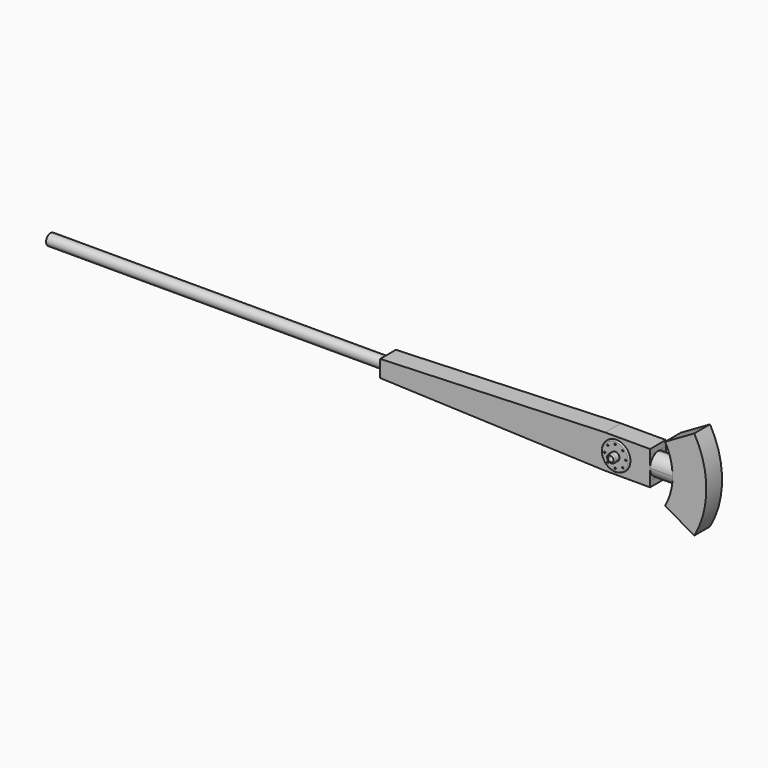
from build123d import *

# Parameters (mm, degrees)
F1_R          = 12.7
F2_DEPTH      = 88.9
F4_DEPTH      = 152.4
F5_R          = 25.4
F5_R_2        = 23.8125
F6_DEPTH      = 1524
F7_R          = 63.5
F7_R_2        = 3.175
F7_R_3        = 12.7
F8_DEPTH      = 6.35
F9_R          = 19.05
F9_R_2        = 12.7
F10_DEPTH     = 25.4
F11_R         = 5.08
F12_R         = 63.5
F12_R_2       = 3.175
F12_R_3       = 12.7
F13_DEPTH     = 6.35
F14_R         = 19.05
F14_R_2       = 12.7
F15_DEPTH     = 25.4
F16_R         = 5.08
F17_T4_DEPTH  = 222.8331578668
F17_S5_R      = 254
F17_T6_DEPTH  = 119
F17_T10_DEPTH = 222.8331578668
F17_S11_R     = 254
F17_T12_DEPTH = 119
F17_T16_DEPTH = 222.8331578668
F17_S17_R     = 254
F17_T18_DEPTH = 119
F17_T22_DEPTH = 222.8331578668
F17_S23_R     = 254
F17_T24_DEPTH = 119


# Not quite as in the source:
# - a fillet or chamfer that OpenCascade refuses, or shapes differently, is made with other operations: its cross-section is extruded or revolved along the edge and cut away or added


with BuildPart() as f2:
    # F1 (on Front) → F2 (new body)
    with BuildSketch(Plane.XZ):
        with BuildLine():
            Line((0, 76.2), (0, -76.2))
            Line((0, -76.2), (1219.2, -76.2))
            Line((1219.2, -76.2), (1219.2, -50.8))
            Line((1219.2, -50.8), (1315.6681578668, -50.8))
            ThreePointArc((1315.6681578668, -50.8), (1304.2953066, -90.0665273172), (1286.7704525612, -127))
            Line((1286.7704525612, -127), (1418.752724098, -203.2))
            ThreePointArc((1418.752724098, -203.2), (1473.2, 0), (1418.752724098, 203.2))
            Line((1418.752724098, 203.2), (1286.7704525612, 127))
            ThreePointArc((1286.7704525612, 127), (1304.2953066, 90.0665273172), (1315.6681578668, 50.8))
            Line((1315.6681578668, 50.8), (1219.2, 50.8))
            Line((1219.2, 50.8), (1219.2, 76.2))
            Line((1219.2, 76.2), (0, 76.2))
        make_face()
        with Locations((1066.8, 0)):
            Circle(F1_R, mode=Mode.SUBTRACT)
    extrude(amount=F2_DEPTH)

    # F3 (on face) → F4 (cut)
    with BuildSketch(Plane.XZ.offset(88.9)):
        Polygon((1016, 76.2), (0, 76.2), (0, 38.1), align=None)
        Polygon((0, -38.1), (0, -76.2), (1016, -76.2), align=None)
    extrude(amount=-F4_DEPTH, mode=Mode.SUBTRACT)

    # F5 (on face) → F6 (join)
    with BuildSketch(Plane(origin=(0, 0, 0), x_dir=(0, -1, 0), z_dir=(-1, 0, 0))):
        with Locations((44.45, 0)):
            Circle(F5_R)
        with Locations((44.45, 0)):
            Circle(F5_R_2, mode=Mode.SUBTRACT)
    extrude(amount=F6_DEPTH)

    # F7 (on face) → F8 (join)
    with BuildSketch(Plane.XZ.offset(88.9)):
        with Locations((1066.8, 0)):
            Circle(F7_R)
        with Locations((1033.124039546, -33.675960454)):
            Circle(F7_R_2, mode=Mode.SUBTRACT)
        with Locations((1066.8, -47.625)):
            Circle(F7_R_2, mode=Mode.SUBTRACT)
        with Locations((1100.475960454, -33.675960454)):
            Circle(F7_R_2, mode=Mode.SUBTRACT)
        with Locations((1019.175, 0)):
            Circle(F7_R_2, mode=Mode.SUBTRACT)
        with Locations((1033.124039546, 33.675960454)):
            Circle(F7_R_2, mode=Mode.SUBTRACT)
        with Locations((1066.8, 0)):
            Circle(F7_R_3, mode=Mode.SUBTRACT)
        with Locations((1114.425, 0)):
            Circle(F7_R_2, mode=Mode.SUBTRACT)
        with Locations((1066.8, 47.625)):
            Circle(F7_R_2, mode=Mode.SUBTRACT)
        with Locations((1100.475960454, 33.675960454)):
            Circle(F7_R_2, mode=Mode.SUBTRACT)
    extrude(amount=F8_DEPTH)

    # F9 (on face) → F10 (join)
    with BuildSketch(Plane.XZ.offset(95.25)):
        with Locations((1066.8, 0)):
            Circle(F9_R)
        with Locations((1066.8, 0)):
            Circle(F9_R_2, mode=Mode.SUBTRACT)
    extrude(amount=F10_DEPTH)

    # F11
    f11_edges = [f2.edges().sort_by_distance(p)[0] for p in [
        (1047.75, -120.65, 0),
        (1003.3, -95.25, 0),
    ]]
    fillet(f11_edges, radius=F11_R)

    # F12 (on face) → F13 (join)
    with BuildSketch(Plane(origin=(0, 0, 0), x_dir=(-1, 0, 0), z_dir=(0, 1, 0))):
        with Locations((-1066.8, 0)):
            Circle(F12_R)
        with Locations((-1100.475960454, -33.675960454)):
            Circle(F12_R_2, mode=Mode.SUBTRACT)
        with Locations((-1066.8, -47.625)):
            Circle(F12_R_2, mode=Mode.SUBTRACT)
        with Locations((-1033.124039546, -33.675960454)):
            Circle(F12_R_2, mode=Mode.SUBTRACT)
        with Locations((-1114.425, 0)):
            Circle(F12_R_2, mode=Mode.SUBTRACT)
        with Locations((-1100.475960454, 33.675960454)):
            Circle(F12_R_2, mode=Mode.SUBTRACT)
        with Locations((-1066.8, 0)):
            Circle(F12_R_3, mode=Mode.SUBTRACT)
        with Locations((-1019.175, 0)):
            Circle(F12_R_2, mode=Mode.SUBTRACT)
        with Locations((-1066.8, 47.625)):
            Circle(F12_R_2, mode=Mode.SUBTRACT)
        with Locations((-1033.124039546, 33.675960454)):
            Circle(F12_R_2, mode=Mode.SUBTRACT)
    extrude(amount=F13_DEPTH)

    # F14 (on face) → F15 (join)
    with BuildSketch(Plane(origin=(0, 6.35, 0), x_dir=(-1, 0, 0), z_dir=(0, 1, 0))):
        with Locations((-1066.8, 0)):
            Circle(F14_R)
        with Locations((-1066.8, 0)):
            Circle(F14_R_2, mode=Mode.SUBTRACT)
    extrude(amount=F15_DEPTH)

    # F16
    f16_edges = [f2.edges().sort_by_distance(p)[0] for p in [
        (1130.3, 6.35, 0),
        (1085.85, 31.75, 0),
    ]]
    fillet(f16_edges, radius=F16_R)

    # F17: fillet of radius 50.546 on 4 edges, made by hand


with BuildPart() as f17_tool2:
    # F17_s3 → F17_t4 (new body)
    with BuildSketch(Plane.YZ.offset(1442.0331578668)):
        with BuildLine():
            ThreePointArc((-38.354, 50.8), (-74.0954193619, 35.9954193619), (-88.9, 0.254))
            Line((-88.9, 0.254), (-88.9, 50.8))
            Line((-88.9, 50.8), (-38.354, 50.8))
        make_face()
    extrude(amount=-F17_T4_DEPTH)

    # F17_s5 → F17_t6 (intersect, symmetric)
    with BuildSketch(Plane.XZ.offset(63.6)):
        with Locations((1066.8, 0)):
            Circle(F17_S5_R)
    extrude(amount=F17_T6_DEPTH, both=True, mode=Mode.INTERSECT)


with BuildPart() as f2_1:
    add(f2.part)

    # F17_t1: cut F17_tool2
    add(f17_tool2.part, mode=Mode.SUBTRACT)


with BuildPart() as f17_tool8:
    # F17_s9 → F17_t10 (new body)
    with BuildSketch(Plane.YZ.offset(1219.2)):
        with BuildLine():
            ThreePointArc((-38.354, -50.8), (-74.0954193619, -35.9954193619), (-88.9, -0.254))
            Line((-88.9, -0.254), (-88.9, -50.8))
            Line((-88.9, -50.8), (-38.354, -50.8))
        make_face()
    extrude(amount=F17_T10_DEPTH)

    # F17_s11 → F17_t12 (intersect, symmetric)
    with BuildSketch(Plane.XZ.offset(63.6)):
        with Locations((1066.8, 0)):
            Circle(F17_S11_R)
    extrude(amount=F17_T12_DEPTH, both=True, mode=Mode.INTERSECT)


with BuildPart() as f2_2:
    add(f2_1.part)

    # F17_t7: cut F17_tool8
    add(f17_tool8.part, mode=Mode.SUBTRACT)


with BuildPart() as f17_tool14:
    # F17_s15 → F17_t16 (new body)
    with BuildSketch(Plane.YZ.offset(1219.2)):
        with BuildLine():
            ThreePointArc((0, -0.254), (-14.8045806381, -35.9954193619), (-50.546, -50.8))
            Line((-50.546, -50.8), (0, -50.8))
            Line((0, -50.8), (0, -0.254))
        make_face()
    extrude(amount=F17_T16_DEPTH)

    # F17_s17 → F17_t18 (intersect, symmetric)
    with BuildSketch(Plane.XZ.offset(25.3)):
        with Locations((1066.8, 0)):
            Circle(F17_S17_R)
    extrude(amount=F17_T18_DEPTH, both=True, mode=Mode.INTERSECT)


with BuildPart() as f2_3:
    add(f2_2.part)

    # F17_t13: cut F17_tool14
    add(f17_tool14.part, mode=Mode.SUBTRACT)


with BuildPart() as f17_tool20:
    # F17_s21 → F17_t22 (new body)
    with BuildSketch(Plane.YZ.offset(1442.0331578668)):
        with BuildLine():
            ThreePointArc((0, 0.254), (-14.8045806381, 35.9954193619), (-50.546, 50.8))
            Line((-50.546, 50.8), (0, 50.8))
            Line((0, 50.8), (0, 0.254))
        make_face()
    extrude(amount=-F17_T22_DEPTH)

    # F17_s23 → F17_t24 (intersect, symmetric)
    with BuildSketch(Plane.XZ.offset(25.3)):
        with Locations((1066.8, 0)):
            Circle(F17_S23_R)
    extrude(amount=F17_T24_DEPTH, both=True, mode=Mode.INTERSECT)


with BuildPart() as f2_4:
    add(f2_3.part)

    # F17_t19: cut F17_tool20
    add(f17_tool20.part, mode=Mode.SUBTRACT)


solid = f2_4.part
